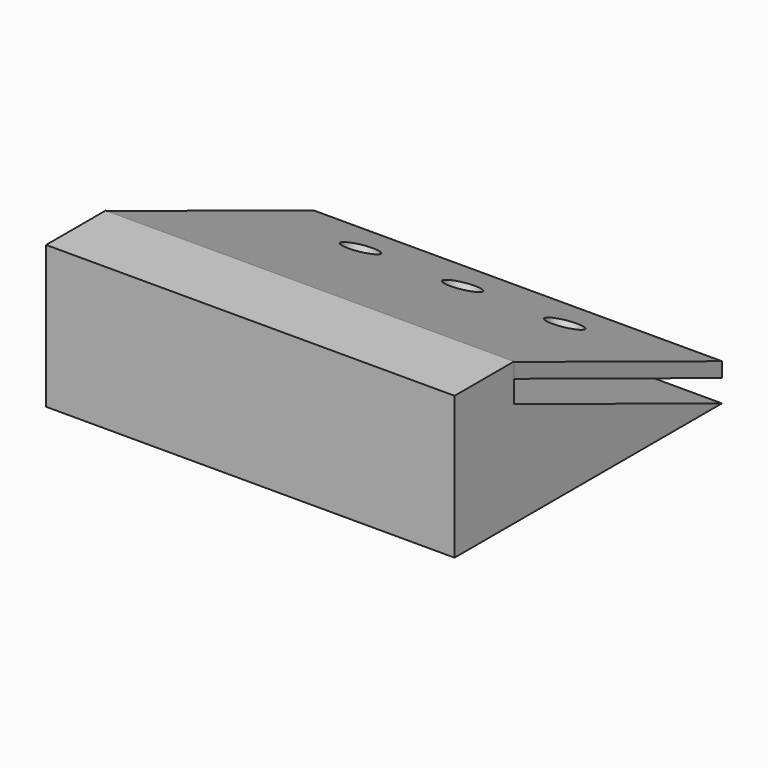
from build123d import *

# Parameters (mm, degrees)
F1_DEPTH = 55
F5_DEPTH = 55
F6_W     = 55
F6_H     = 19.191428078
F7_DEPTH = 10
F8_R     = 2.25
F9_DEPTH = 25


with BuildPart() as f1:
    # F0 (on Right) → F1 (new body)
    with BuildSketch(Plane.YZ):
        Polygon((24.9822678417, 0), (-10.0177321583, 14.1409179042), (-10.0177321583, 0), align=None)
    extrude(amount=F1_DEPTH)

    # F6 (on face) → F7 (join)
    with BuildSketch(Plane.XZ.offset(10.0177321583)):
        with Locations((27.5, 9.595714039)):
            Rectangle(F6_W, F6_H)
    extrude(amount=F7_DEPTH)


with BuildPart() as f5:
    # F4 (on face) → F5 (new body)
    with BuildSketch(Plane.YZ.offset(55)):
        Polygon((-10.016492568, 19.1397086233), (-10.016492568, 17.1397086233), (24.9822754413, 2.9999588151), (24.9822754413, 4.9999588151), align=None)
    extrude(amount=-F5_DEPTH)

    # F8 (on face) → F9 (cut)
    with BuildSketch(Plane(origin=(0, 5.242051865, 12.9751487547), x_dir=(1, 0, 0), z_dir=(0, 0.3745913268, 0.9271900225))):
        with Locations((13.75, 11.2903753235)):
            Circle(F8_R)
        with BuildLine():
            ThreePointArc((25.25, 11.2903753235), (27.5, 9.0403753235), (29.75, 11.2903753235))
            Line((29.75, 11.2903753235), (27.5, 11.2903753235))
            Line((27.5, 11.2903753235), (25.25, 11.2903753235))
        make_face()
        with BuildLine():
            Line((27.5, 11.2903753235), (29.75, 11.2903753235))
            ThreePointArc((29.75, 11.2903753235), (27.5, 13.5403753235), (25.25, 11.2903753235))
            Line((25.25, 11.2903753235), (27.5, 11.2903753235))
        make_face()
        with BuildLine():
            ThreePointArc((43.5, 11.2903753235), (41.25, 13.5403753235), (39, 11.2903753235))
            ThreePointArc((39, 11.2903753235), (41.25, 9.0403753235), (43.5, 11.2903753235))
        make_face()
    extrude(amount=-F9_DEPTH, mode=Mode.SUBTRACT)


solid = Compound([f1.part, f5.part])
